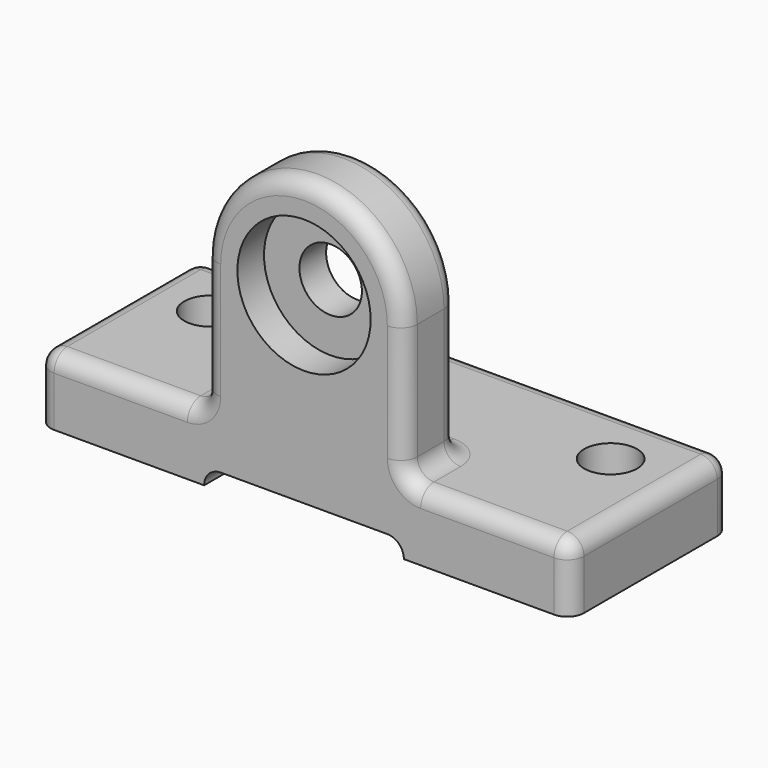
from build123d import *

# Parameters (mm, degrees)
F0_W           = 101.6
F0_H           = 38.1
F1_DEPTH       = 12.7
F2_W           = 38.1
F2_H           = 12.7
F3_DEPTH       = 12.7
F4_D           = 11.90625
F4_CBORE_D     = 25.4
F4_CBORE_DEPTH = 6.35
F5_W           = 38.0556955934
F5_H           = 3.175
F6_DEPTH       = 38.101
F8_D           = 10.0838
F9_R           = 3.17499
F10_R          = 3.17499


# Not quite as in the source:
# - a fillet or chamfer is up to 0.001 mm smaller than in the source, because OpenCascade refuses the exact size
# - a length typed as a fraction of an inch, garbled in the dataset ("3 / 203.2 mm" for 3/8 in), is restored


with BuildPart() as f1:
    # F0 (on Top) → F1 (new body)
    with BuildSketch(Plane.XY):
        with Locations((50.8, 19.05)):
            Rectangle(F0_W, F0_H)
    extrude(amount=F1_DEPTH)

    # F2 (on face) → F3 (join)
    with BuildSketch(Plane.XZ):
        with BuildLine():
            Line((31.75, 38.1), (31.75, 12.7))
            Line((31.75, 12.7), (69.85, 12.7))
            Line((69.85, 12.7), (69.85, 38.1))
            ThreePointArc((69.85, 38.1), (50.8, 57.15), (31.75, 38.1))
        make_face()
        with Locations((50.8, 6.35)):
            Rectangle(F2_W, F2_H)
    extrude(amount=-F3_DEPTH)

    # F4 (through all)
    with Locations(Plane.XZ):
        with Locations((50.8, 38.1)):
            CounterBoreHole(F4_D / 2, F4_CBORE_D / 2, F4_CBORE_DEPTH)

    # F5 (on face) → F6 (cut, through all)
    with BuildSketch(Plane(origin=(0, 38.1, 0), x_dir=(-1, 0, 0), z_dir=(0, 1, 0))):
        with Locations((-50.798330456, 1.5875)):
            Rectangle(F5_W, F5_H)
    extrude(amount=-F6_DEPTH, mode=Mode.SUBTRACT)

    # F8 (through all)
    with Locations(Plane.XY.offset(12.7)):
        with Locations((12.7, 25.4), (88.9, 25.4)):
            Hole(F8_D / 2)

    # F9 (radius 3.175 in the source; OpenCascade refuses exactly that, so slightly less here)
    f9_edges = [f1.edges().sort_by_distance(p)[0] for p in [
        (101.6, 38.1, 6.35),
        (0, 38.1, 6.35),
        (0, 0, 6.35),
        (101.6, 0, 6.35),
        (31.770483, 19.05, 3.175),
        (69.826178, 19.05, 3.175),
    ]]
    fillet(f9_edges, radius=F9_R)

    # F10 (radius 3.175 in the source; OpenCascade refuses exactly that, so slightly less here)
    f10_edges = [f1.edges().sort_by_distance(p)[0] for p in [
        (17.462495, 0, 12.7),
        (50.8, 38.1, 12.7),
        (0, 19.05, 12.7),
        (84.137505, 0, 12.7),
        (101.6, 19.05, 12.7),
        (69.85, 6.35, 12.7),
        (50.8, 0, 57.15),
        (50.8, 12.7, 57.15),
        (69.85, 12.7, 25.4),
        (50.8, 12.7, 12.7),
        (31.75, 6.35, 12.7),
        (31.75, 12.7, 25.4),
        (31.75, 0, 25.4),
        (69.85, 0, 25.4),
    ]]
    fillet(f10_edges, radius=F10_R)


solid = f1.part
